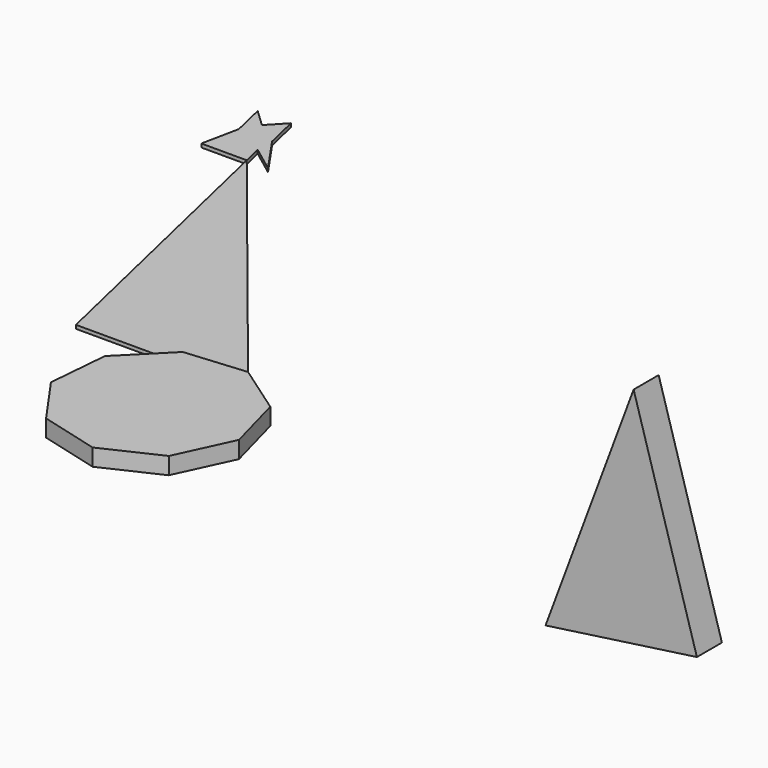
from build123d import *

# Parameters (mm, degrees)
F1_DEPTH = 2.794
F3_DEPTH = 2.032
F6_DEPTH = 1.016
F8_DEPTH = 8.89


# Not quite as in the source:
# - the program builds the solid bodies; features that only make, move or delete a surface that nothing else refers to are left out


with BuildPart() as f1:
    # F0 (on Top) → F1 (new body)
    with BuildSketch(Plane.XY):
        Polygon((-52.5751584309, -42.0525174268), (-45.2585345965, -26.281562852), (-49.7910497594, -9.4972755918), (-64.0518897016, 0.4467898081), (-81.3682489225, -1.1023053687), (-93.6376104928, -13.4197222729), (-95.119003775, -30.7420046421), (-85.1192683885, -44.9638640401), (-68.3173916553, -49.4307343961), align=None)
    extrude(amount=F1_DEPTH)

    # F3 (add): a face of the model
    f3_faces = [f1.faces().sort_by_distance(p)[0] for p in [
        (-70.5820173025, -24.1159107536, 2.794),
    ]]
    extrude(f3_faces, amount=F3_DEPTH)

    # F5 (on Top) → F6 (join)
    with BuildSketch(Plane.XY):
        Polygon((-132.4096173048, 85.4147747159), (-112.612426281, 0), (-63.6733919382, 0), align=None)
    extrude(amount=F6_DEPTH)

    # F5 (on Top) → F6, piece 2 (join)
    with BuildSketch(Plane.XY):
        Polygon((-145.3195103792, 85.4147747159), (-132.4096173048, 85.4147747159), (-133.6767779322, 90.88192606), (-126.3700127602, 85.4147747159), (-133.6767779322, 96.0004851222), (-135.8651248663, 105.4420852036), (-140.3465569019, 100.7212851629), (-145.3195103792, 105.4420852036), (-143.131163445, 96.0004851222), align=None)
    extrude(amount=F6_DEPTH)


with BuildPart() as f8:
    # F7 (on Front) → F8 (new body)
    with BuildSketch(Plane.XZ):
        Polygon((52.9666729271, 42.2895699739), (27.9397200793, -24.8587857932), (70.943787694, -18.7894441187), align=None)
    extrude(amount=F8_DEPTH)


solid = Compound([f1.part, f8.part])
